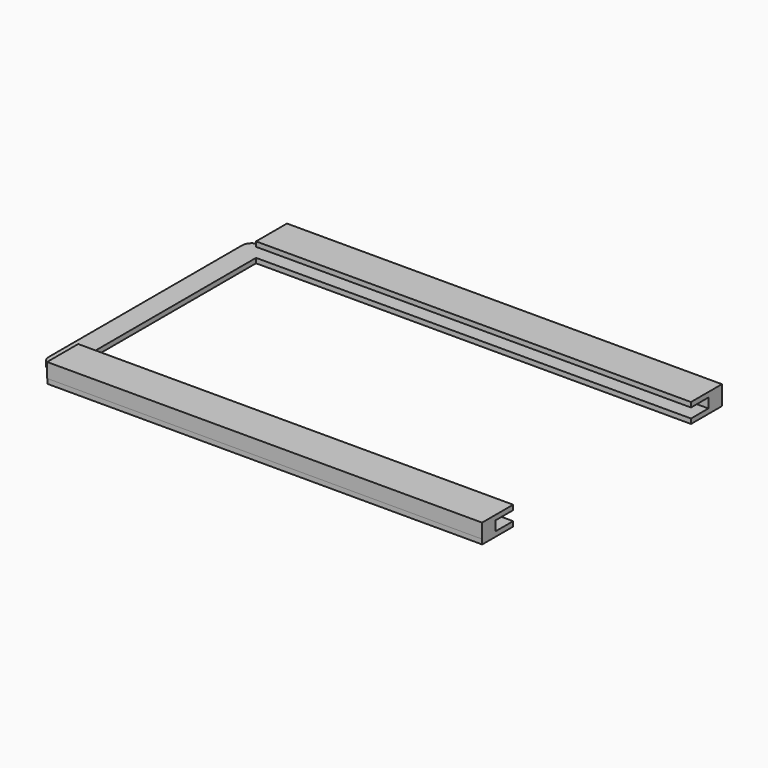
from build123d import *

# Parameters (mm, degrees)
F2_DEPTH = 1
F3_W     = 90
F3_H     = 3.5
F3_H_2   = 0.0419686139
F3_H_3   = 3.4580313861
F4_DEPTH = 2
F5_W     = 90
F5_H     = 3.5
F5_H_2   = 4.5
F5_H_3   = 8.0419686139
F6_DEPTH = 1


# Not quite as in the source:
# - a feature names something its author has since deleted; it is built from what else it names


with BuildPart() as f2:
    # F1 (on face) → F2 (new body)
    with BuildSketch(Plane.XY):
        with BuildLine():
            Line((14.8598281033, 4.21106866), (-75.1401718967, 4.21106866))
            Line((-75.1401718967, 4.21106866), (-75.1401718967, 0.21106866))
            Line((-75.1401718967, 0.21106866), (4.3706398308, 0.21106866))
            ThreePointArc((4.3706398308, 0.21106866), (5.7848533932, -0.3747177776), (6.3706398308, -1.78893134))
            Line((6.3706398308, -1.78893134), (6.3706398308, -3.78893134))
            Line((6.3706398308, -3.78893134), (14.8598281033, -3.78893134))
            Line((14.8598281033, -3.78893134), (14.8598281033, 4.21106866))
        make_face()
        with BuildLine():
            Line((14.8598281033, -49.78893134), (6.3706398308, -49.78893134))
            Line((6.3706398308, -49.78893134), (6.3706398308, -51.78893134))
            ThreePointArc((6.3706398308, -51.78893134), (5.7848533932, -53.2031449024), (4.3706398308, -53.78893134))
            Line((4.3706398308, -53.78893134), (-75.1401718967, -53.78893134))
            Line((-75.1401718967, -53.78893134), (-75.1401718967, -57.78893134))
            Line((-75.1401718967, -57.78893134), (14.8598281033, -57.78893134))
            Line((14.8598281033, -57.78893134), (14.8598281033, -49.78893134))
        make_face()
        with BuildLine():
            Line((-75.1401718967, -3.78893134), (-75.1401718967, 0.21106866))
            Line((-75.1401718967, 0.21106866), (-77.6293601692, 0.21106866))
            ThreePointArc((-77.6293601692, 0.21106866), (-79.0435737315, -0.3747177776), (-79.6293601692, -1.78893134))
            Line((-79.6293601692, -1.78893134), (-79.6293601692, -51.78893134))
            ThreePointArc((-79.6293601692, -51.78893134), (-79.0435737315, -53.2031449024), (-77.6293601692, -53.78893134))
            Line((-77.6293601692, -53.78893134), (-75.1401718967, -53.78893134))
            Line((-75.1401718967, -53.78893134), (-75.1401718967, -49.78893134))
            Line((-75.1401718967, -49.78893134), (-75.1401718967, -3.78893134))
        make_face()
        with BuildLine():
            Line((-68.8141618371, -49.78893134), (-75.1401718967, -49.78893134))
            Line((-75.1401718967, -49.78893134), (-75.1401718967, -53.78893134))
            Line((-75.1401718967, -53.78893134), (4.3706398308, -53.78893134))
            ThreePointArc((4.3706398308, -53.78893134), (5.7848533932, -53.2031449024), (6.3706398308, -51.78893134))
            Line((6.3706398308, -51.78893134), (6.3706398308, -49.78893134))
            Line((6.3706398308, -49.78893134), (6.1858381629, -49.78893134))
            Line((6.1858381629, -49.78893134), (0.4592296318, -49.78893134))
            Line((0.4592296318, -49.78893134), (-68.8141618371, -49.78893134))
        make_face()
        with BuildLine():
            Line((4.3706398308, 0.21106866), (-75.1401718967, 0.21106866))
            Line((-75.1401718967, 0.21106866), (-75.1401718967, -3.78893134))
            Line((-75.1401718967, -3.78893134), (-68.8141618371, -3.78893134))
            Line((-68.8141618371, -3.78893134), (6.1858381629, -3.78893134))
            Line((6.1858381629, -3.78893134), (6.3706398308, -3.78893134))
            Line((6.3706398308, -3.78893134), (6.3706398308, -1.78893134))
            ThreePointArc((6.3706398308, -1.78893134), (5.7848533932, -0.3747177776), (4.3706398308, 0.21106866))
        make_face()
    extrude(amount=F2_DEPTH)

    # F3 (on face) → F4 (join)
    with BuildSketch(Plane.XY.offset(1)):
        with Locations((-30.1401718967, 2.46106866)):
            Rectangle(F3_W, F3_H)
        with Locations((-30.1401718967, -57.8099156469)):
            Rectangle(F3_W, F3_H_2)
        with Locations((-30.1401718967, -56.0599156469)):
            Rectangle(F3_W, F3_H_3)
    extrude(amount=F4_DEPTH)

    # F5 (on face) → F6 (join)
    with BuildSketch(Plane.XY.offset(3)):
        with Locations((-30.1401718967, 2.46106866)):
            Rectangle(F5_W, F5_H)
        with Locations((-30.1401718967, -1.53893134)):
            Rectangle(F5_W, F5_H_2)
        with Locations((-30.1401718967, -53.8099156469)):
            Rectangle(F5_W, F5_H_3)
    extrude(amount=F6_DEPTH)


solid = f2.part
